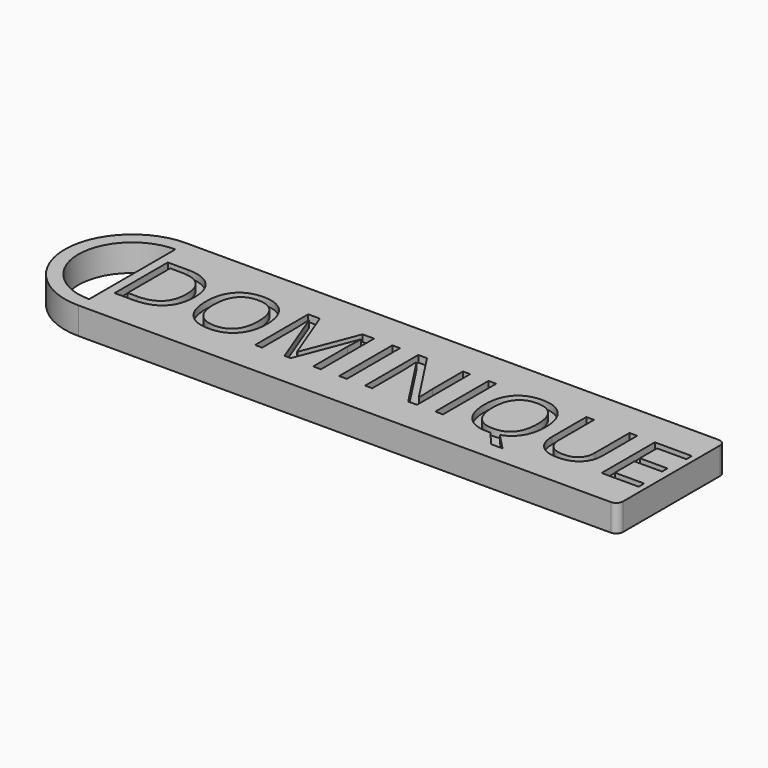
from build123d import *

# Parameters (mm, degrees)
F4_DEPTH     = 2
F1_R         = 0.5
F2_TEXT_SIZE = 6.9088357532
F3_DEPTH     = 0.5


# Not quite as in the source:
# - Text() gives the source's letters only with a copy of the font that has no kerning and outlines rounded to 1/6400 em; it was checked with that copy


with BuildPart() as f4:
    # F0 (on Top) → F4 (new body)
    with BuildSketch(Plane.XY):
        Polygon((34.7291392038, 3.2207785361), (-5.2708607962, 3.2207785361), (-5.2708607962, 2.2207785361), (-5.2708607962, -5.7792214639), (-5.2708607962, -6.7792214639), (34.7291392038, -6.7792214639), align=None)
        with BuildLine():
            Line((-5.2708607962, 2.2207785361), (-5.2708607962, 3.2207785361))
            ThreePointArc((-5.2708607962, 3.2207785361), (-10.2708607962, -1.7792214639), (-5.2708607962, -6.7792214639))
            Line((-5.2708607962, -6.7792214639), (-5.2708607962, -5.7792214639))
            ThreePointArc((-5.2708607962, -5.7792214639), (-9.2708607962, -1.7792214639), (-5.2708607962, 2.2207785361))
        make_face()
    extrude(amount=F4_DEPTH)

    # F1
    f1_edges = [f4.edges().sort_by_distance(p)[0] for p in [
        (34.729139, -6.779221, 1),
        (34.729139, 3.220779, 1),
    ]]
    fillet(f1_edges, radius=F1_R)

    # F2 (on face) → F3 (cut)
    with BuildSketch(Plane.XY.offset(2)):
        with Locations((-5.2708607962, -4.2664023351)):
            Text('DOMINIQUE', F2_TEXT_SIZE, font='Open Sans', text_align=(TextAlign.LEFT, TextAlign.BOTTOM))
    extrude(amount=-F3_DEPTH, mode=Mode.SUBTRACT)


solid = f4.part
